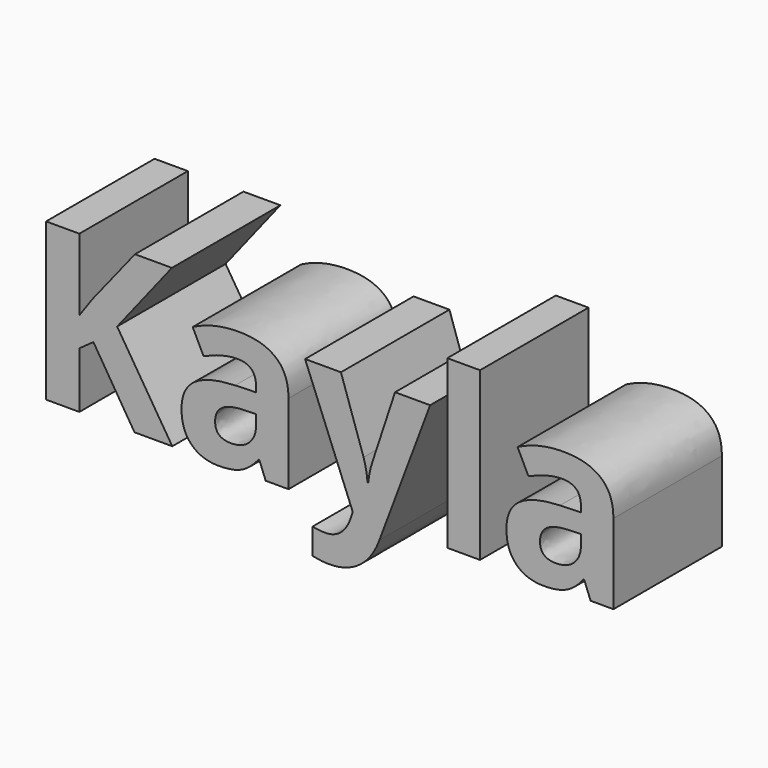
from build123d import *

# Parameters (mm, degrees)
F0_TEXT_SIZE = 41.1722123519
F1_DEPTH     = 25.4


# Not quite as in the source:
# - Text() gives the source's letters only with a copy of the font that has no kerning and outlines rounded to 1/6400 em; it was checked with that copy


with BuildPart() as f1:
    # F0 (on Front) → F1 (new body)
    with BuildSketch(Plane.XZ):
        with Locations((-57.2733421135, 8.3463685587)):
            Text('Kayla', F0_TEXT_SIZE, font='Open Sans', font_style=FontStyle.BOLD, text_align=(TextAlign.LEFT, TextAlign.BOTTOM))
    extrude(amount=F1_DEPTH)


solid = f1.part
